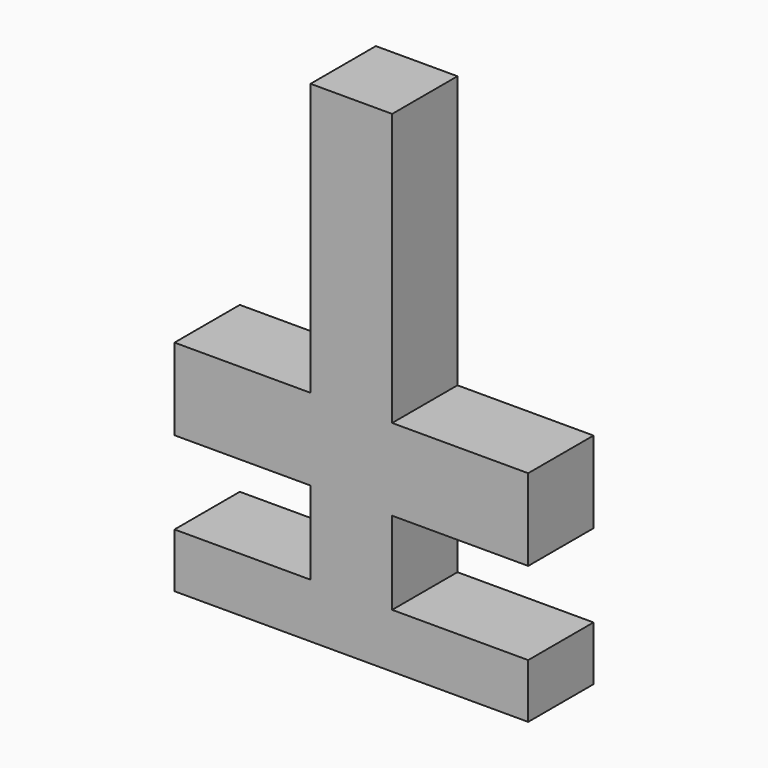
from build123d import *

# Parameters (mm, degrees)
F0_W     = 19.05
F0_H     = 38.6983451158
F0_H_2   = 127
F0_H_3   = 1.5088043451
F1_DEPTH = 38.1


with BuildPart() as f1:
    # F0 (on Front) → F1 (new body)
    with BuildSketch(Plane.XZ):
        Polygon((82.55, -83.5251413941), (19.05, -83.5251413941), (19.05, -85.0339457393), (0, -85.0339457393), (0, -108.9251413941), (82.55, -108.9251413941), align=None)
        Polygon((0, -44.8267962784), (0, -6.7267962784), (-19.05, -6.7267962784), (-82.55, -6.7267962784), (-82.55, -44.8267962784), (-19.05, -44.8267962784), align=None)
        Polygon((19.05, -6.7267962784), (0, -6.7267962784), (0, -44.8267962784), (19.05, -44.8267962784), (82.55, -44.8267962784), (82.55, -6.7267962784), align=None)
        with Locations((9.525, -64.1759688362)):
            Rectangle(F0_W, F0_H)
        with Locations((-9.525, -64.1759688362)):
            Rectangle(F0_W, F0_H)
        with Locations((9.525, 56.7732037216)):
            Rectangle(F0_W, F0_H_2)
        Polygon((0, -85.0339457393), (0, -83.5251413941), (-19.05, -83.5251413941), (-82.55, -83.5251413941), (-82.55, -108.9251413941), (0, -108.9251413941), align=None)
        with Locations((-9.525, 56.7732037216)):
            Rectangle(F0_W, F0_H_2)
        with Locations((9.525, -84.2795435667)):
            Rectangle(F0_W, F0_H_3)
    extrude(amount=F1_DEPTH)


solid = f1.part
